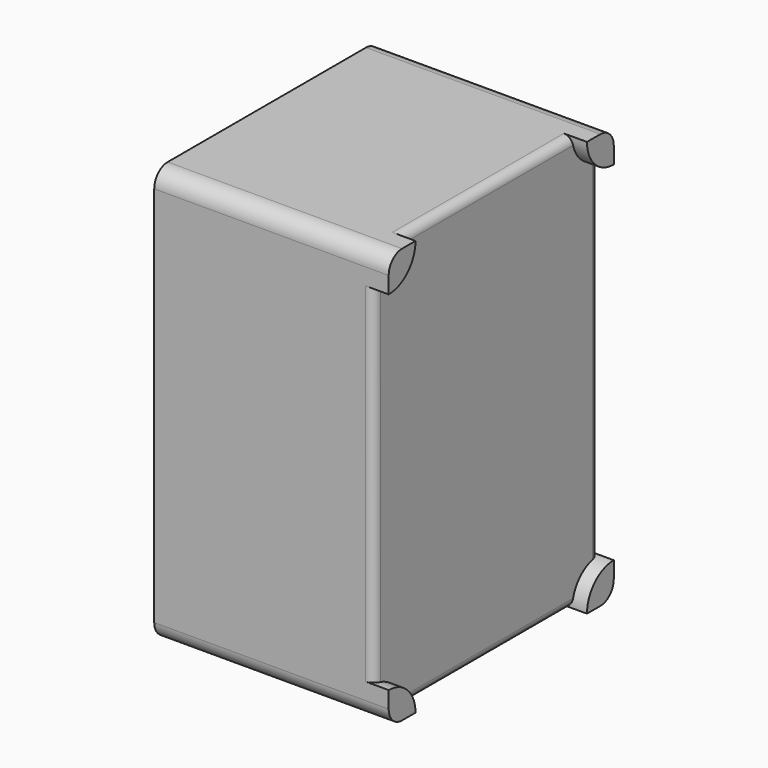
from build123d import *

# Parameters (mm, degrees)
F1_DEPTH = 1.524
F3_DEPTH = 40.132
F5_DEPTH = 2.794
F8_R     = 1.5875
F9_R     = 1.5875
F10_R    = 1.5875
F11_R    = 1.5875


with BuildPart() as f1:
    # F0 (on Right) → F1 (new body)
    with BuildSketch(Plane.YZ):
        with BuildLine():
            ThreePointArc((26.67, 36.195), (25.7400640303, 38.4400640303), (23.495, 39.37))
            Line((23.495, 39.37), (-23.495, 39.37))
            ThreePointArc((-23.495, 39.37), (-25.7400640303, 38.4400640303), (-26.67, 36.195))
            Line((-26.67, 36.195), (-26.67, -36.195))
            ThreePointArc((-26.67, -36.195), (-25.7400640303, -38.4400640303), (-23.495, -39.37))
            Line((-23.495, -39.37), (23.495, -39.37))
            ThreePointArc((23.495, -39.37), (25.7400640303, -38.4400640303), (26.67, -36.195))
            Line((26.67, -36.195), (26.67, 36.195))
        make_face()
    extrude(amount=F1_DEPTH)

    # F2 (on face) → F3 (join)
    with BuildSketch(Plane(origin=(0, 0, 0), x_dir=(0, -1, 0), z_dir=(-1, 0, 0))):
        with BuildLine():
            Line((23.495, 39.37), (-23.495, 39.37))
            ThreePointArc((-23.495, 39.37), (-25.7400640303, 38.4400640303), (-26.67, 36.195))
            Line((-26.67, 36.195), (-26.67, -36.195))
            ThreePointArc((-26.67, -36.195), (-25.7400640303, -38.4400640303), (-23.495, -39.37))
            Line((-23.495, -39.37), (23.495, -39.37))
            ThreePointArc((23.495, -39.37), (25.7400640303, -38.4400640303), (26.67, -36.195))
            Line((26.67, -36.195), (26.67, 36.195))
            ThreePointArc((26.67, 36.195), (25.7400640303, 38.4400640303), (23.495, 39.37))
        make_face()
        with BuildLine():
            ThreePointArc((25.146, -36.2585), (24.6810320151, -37.3810320151), (23.5585, -37.846))
            Line((23.5585, -37.846), (-23.5585, -37.846))
            ThreePointArc((-23.5585, -37.846), (-24.6810320151, -37.3810320151), (-25.146, -36.2585))
            Line((-25.146, -36.2585), (-25.146, 36.2585))
            ThreePointArc((-25.146, 36.2585), (-24.6810320151, 37.3810320151), (-23.5585, 37.846))
            Line((-23.5585, 37.846), (23.5585, 37.846))
            ThreePointArc((23.5585, 37.846), (24.6810320151, 37.3810320151), (25.146, 36.2585))
            Line((25.146, 36.2585), (25.146, -36.2585))
        make_face(mode=Mode.SUBTRACT)
    extrude(amount=F3_DEPTH)

    # F4 (on face) → F5 (join)
    with BuildSketch(Plane.YZ.offset(1.524)):
        with BuildLine():
            ThreePointArc((-26.67, 33.02), (-22.1798719395, 34.8798719395), (-20.32, 39.37))
            Line((-20.32, 39.37), (-23.495, 39.37))
            ThreePointArc((-23.495, 39.37), (-25.7400640303, 38.4400640303), (-26.67, 36.195))
            Line((-26.67, 36.195), (-26.67, 33.02))
        make_face()
    extrude(amount=F5_DEPTH)


with BuildPart() as f6_1:
    # F6: instance of F1
    add(f1.part.mirror(Plane.XY))


with BuildPart() as f1_1:
    add(f1.part)

    add(f6_1.part)  # F7 merges F6_1
    # F7: F6_1, F1 across plane
    add(f6_1.part.mirror(Plane.XZ))
    add(f1.part.mirror(Plane.XZ))

    # F8
    f8_edges = [f1_1.edges().sort_by_distance(p)[0] for p in [
        (1.524, -26.67, 0),
    ]]
    fillet(f8_edges, radius=F8_R)

    # F9
    f9_edges = [f1_1.edges().sort_by_distance(p)[0] for p in [
        (1.524, 0, -39.37),
    ]]
    fillet(f9_edges, radius=F9_R)

    # F10
    f10_edges = [f1_1.edges().sort_by_distance(p)[0] for p in [
        (1.524, 26.67, 0),
    ]]
    fillet(f10_edges, radius=F10_R)

    # F11
    f11_edges = [f1_1.edges().sort_by_distance(p)[0] for p in [
        (1.524, 0, 39.37),
    ]]
    fillet(f11_edges, radius=F11_R)


solid = f1_1.part
